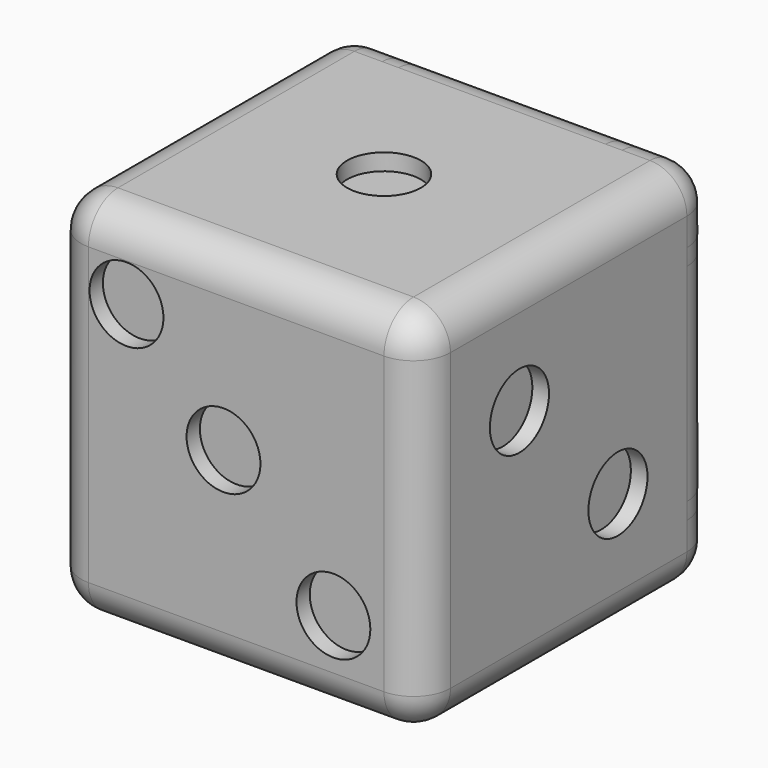
from build123d import *

# Parameters (mm, degrees)
F0_W      = 20
F0_H      = 20
F1_DEPTH  = 20
F5_R      = 2
F8_DEPTH  = 0.9
F2_R      = 2
F9_DEPTH  = 0.9
F4_R      = 2
F10_DEPTH = 0.9
F7_R      = 2
F11_DEPTH = 0.9
F12_DEPTH = 0.9
F3_R      = 2
F13_DEPTH = 0.9
F14_R     = 1.99999


# Not quite as in the source:
# - a fillet or chamfer is up to 0.001 mm smaller than in the source, because OpenCascade refuses the exact size


with BuildPart() as f1:
    # F0 (on Top) → F1 (new body)
    with BuildSketch(Plane.XY):
        with Locations((10, 10)):
            Rectangle(F0_W, F0_H)
    extrude(amount=F1_DEPTH)

    # F5 (on face) → F8 (cut)
    with BuildSketch(Plane(origin=(0, 0, 0), x_dir=(0, -1, 0), z_dir=(-1, 0, 0))):
        with Locations((-16, 16)):
            Circle(F5_R)
        with Locations((-10, 10)):
            Circle(F5_R)
        with Locations((-4, 16)):
            Circle(F5_R)
        with Locations((-4, 4)):
            Circle(F5_R)
        with Locations((-16, 4)):
            Circle(F5_R)
    extrude(amount=-F8_DEPTH, mode=Mode.SUBTRACT)

    # F2 (on face) → F9 (cut)
    with BuildSketch(Plane.XY.offset(20)):
        with Locations((10, 10)):
            Circle(F2_R)
    extrude(amount=-F9_DEPTH, mode=Mode.SUBTRACT)

    # F4 (on face) → F10 (cut)
    with BuildSketch(Plane.YZ.offset(20)):
        with Locations((13.3333333333, 6.6666666667)):
            Circle(F4_R)
        with Locations((6.6666666667, 13.3333333333)):
            Circle(F4_R)
    extrude(amount=-F10_DEPTH, mode=Mode.SUBTRACT)

    # F7 (on face) → F11 (cut)
    with BuildSketch(Plane(origin=(0, 20, 0), x_dir=(-1, 0, 0), z_dir=(0, 1, 0))):
        with Locations((-3.9495522901, 16.0504477099)):
            Circle(F7_R)
        with Locations((-3.9495522901, 3.9495522901)):
            Circle(F7_R)
        with Locations((-16.0504477099, 3.9495522901)):
            Circle(F7_R)
        with Locations((-16.0504477099, 16.0504477099)):
            Circle(F7_R)
    extrude(amount=-F11_DEPTH, mode=Mode.SUBTRACT)

    # F6 (on face) → F12 (cut)
    with BuildSketch(Plane.XZ):
        with BuildLine():
            Line((15.2621462241, 4.7378537759), (13.8479326617, 6.1520673383))
            ThreePointArc((13.8479326617, 6.1520673383), (13.8479326617, 3.3236402136), (16.6763597864, 3.3236402136))
            Line((16.6763597864, 3.3236402136), (15.2621462241, 4.7378537759))
        make_face()
        with BuildLine():
            ThreePointArc((17.2621462241, 4.7378537759), (16.0275130888, 6.585612841), (13.8479326617, 6.1520673383))
            Line((13.8479326617, 6.1520673383), (15.2621462241, 4.7378537759))
            Line((15.2621462241, 4.7378537759), (16.6763597864, 3.3236402136))
            ThreePointArc((16.6763597864, 3.3236402136), (17.1099052891, 3.9724869112), (17.2621462241, 4.7378537759))
        make_face()
        with BuildLine():
            ThreePointArc((11.3126059573, 10.6873940427), (10.077972822, 12.5351531078), (7.8983923949, 12.1016076051))
            Line((7.8983923949, 12.1016076051), (9.3126059573, 10.6873940427))
            Line((9.3126059573, 10.6873940427), (10.7268195196, 9.2731804804))
            ThreePointArc((10.7268195196, 9.2731804804), (11.1603650223, 9.922027178), (11.3126059573, 10.6873940427))
        make_face()
        with BuildLine():
            Line((9.3126059573, 10.6873940427), (7.8983923949, 12.1016076051))
            ThreePointArc((7.8983923949, 12.1016076051), (7.8983923949, 9.2731804804), (10.7268195196, 9.2731804804))
            Line((10.7268195196, 9.2731804804), (9.3126059573, 10.6873940427))
        make_face()
        with BuildLine():
            ThreePointArc((5.475499908, 14.524500092), (5.9090454106, 15.1733467897), (6.0612863456, 15.9387136544))
            ThreePointArc((6.0612863456, 15.9387136544), (4.8266532103, 17.7864727194), (2.6470727832, 17.3529272168))
            Line((2.6470727832, 17.3529272168), (4.0612863456, 15.9387136544))
            Line((4.0612863456, 15.9387136544), (5.475499908, 14.524500092))
        make_face()
        with BuildLine():
            Line((4.0612863456, 15.9387136544), (2.6470727832, 17.3529272168))
            ThreePointArc((2.6470727832, 17.3529272168), (2.6470727832, 14.524500092), (5.475499908, 14.524500092))
            Line((5.475499908, 14.524500092), (4.0612863456, 15.9387136544))
        make_face()
    extrude(amount=-F12_DEPTH, mode=Mode.SUBTRACT)

    # F3 (on face) → F13 (cut)
    with BuildSketch(Plane(origin=(0, 0, 0), x_dir=(1, 0, 0), z_dir=(0, 0, -1))):
        with Locations((15.949013711, -4.050986289)):
            Circle(F3_R)
        with Locations((15.949013711, -10)):
            Circle(F3_R)
        with Locations((15.949013711, -15.949013711)):
            Circle(F3_R)
        with Locations((4.050986289, -4.050986289)):
            Circle(F3_R)
        with Locations((4.050986289, -10)):
            Circle(F3_R)
        with Locations((4.050986289, -15.949013711)):
            Circle(F3_R)
    extrude(amount=-F13_DEPTH, mode=Mode.SUBTRACT)

    # F14 (radius 2 in the source; OpenCascade refuses exactly that, so slightly less here)
    f14_edges = [f1.edges().sort_by_distance(p)[0] for p in [
        (20, 10, 0),
        (10, 20, 0),
        (0, 20, 10),
        (0, 10, 20),
        (10, 20, 20),
        (20, 10, 20),
        (20, 0, 10),
        (10, 0, 20),
        (20, 20, 10),
        (0, 10, 0),
        (0, 0, 10),
        (10, 0, 0),
    ]]
    fillet(f14_edges, radius=F14_R)


solid = f1.part
